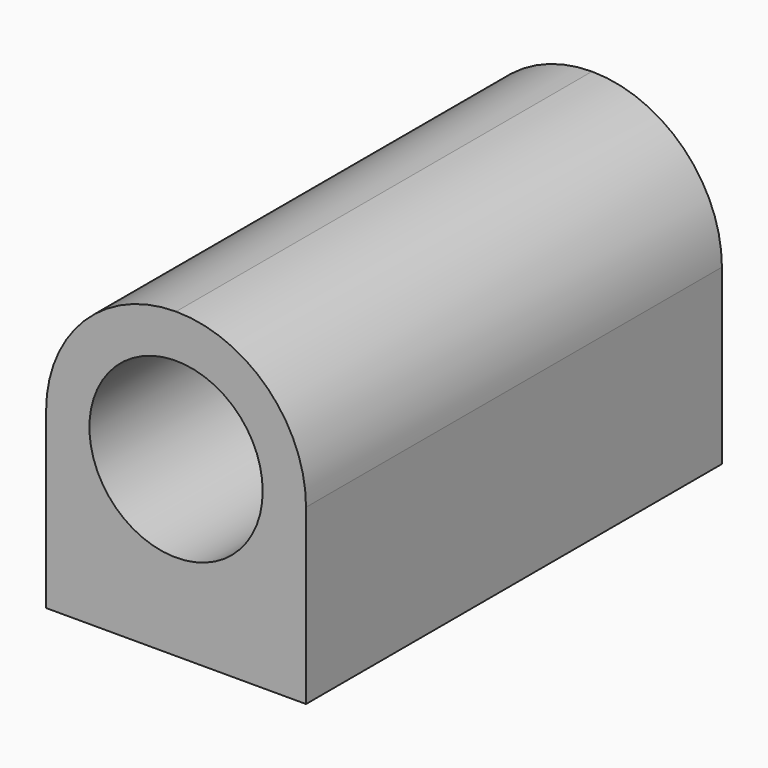
from build123d import *

# Parameters (mm, degrees)
F0_W     = 38.1
F0_H     = 44.45
F1_DEPTH = 76.2
F2_R     = 19.04999
F3_R     = 12.7
F4_DEPTH = 76.201
F5_R     = 1.651
F6_DEPTH = 12.7


# Not quite as in the source:
# - a fillet or chamfer is up to 0.001 mm smaller than in the source, because OpenCascade refuses the exact size


with BuildPart() as f1:
    # F0 (on Front) → F1 (new body)
    with BuildSketch(Plane.XZ):
        with Locations((19.05, 22.225)):
            Rectangle(F0_W, F0_H)
    extrude(amount=F1_DEPTH)

    # F2 (radius 19.05 in the source; OpenCascade refuses exactly that, so slightly less here)
    f2_edges = [f1.edges().sort_by_distance(p)[0] for p in [
        (0, -38.1, 44.45),
        (38.1, -38.1, 44.45),
    ]]
    fillet(f2_edges, radius=F2_R)

    # F3 (on face) → F4 (cut, through all)
    with BuildSketch(Plane.XZ.offset(76.2)):
        with Locations((19.05, 25.4)):
            Circle(F3_R)
    extrude(amount=-F4_DEPTH, mode=Mode.SUBTRACT)

    # F5 (on face) → F6 (cut)
    with BuildSketch(Plane(origin=(0, 0, 0), x_dir=(1, 0, 0), z_dir=(0, 0, -1))):
        with Locations((31.75, 69.85)):
            Circle(F5_R)
        with Locations((6.35, 69.85)):
            Circle(F5_R)
        with Locations((31.75, 6.35)):
            Circle(F5_R)
        with Locations((6.35, 6.35)):
            Circle(F5_R)
    extrude(amount=-F6_DEPTH, mode=Mode.SUBTRACT)


solid = f1.part
